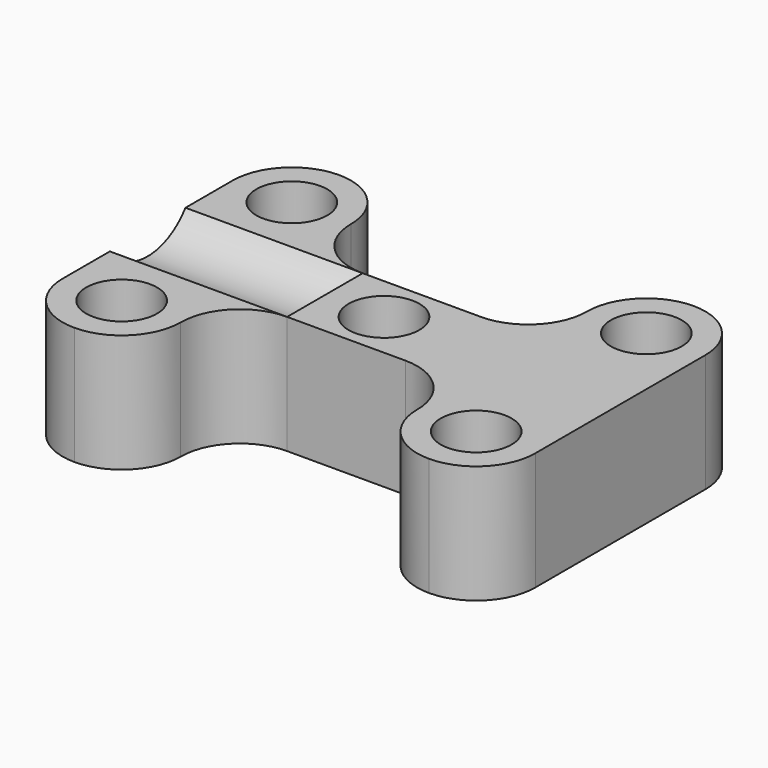
from build123d import *

# Parameters (mm, degrees)
F1_W       = 10
F1_H       = 10
F2_DEPTH   = 10
F1_H_2     = 8
F1_W_2     = 20
F3_DEPTH   = 10
F5_DEPTH   = 15
F6_D       = 6
F6_DEPTH   = 20
F6_TIP     = 1.8025818571
F6_2_D     = 6
F6_2_DEPTH = 20
F6_2_TIP   = 1.8025818571
F6_3_D     = 6
F6_3_DEPTH = 20
F6_3_TIP   = 1.8025818571
F6_4_D     = 6
F6_4_DEPTH = 20
F6_4_TIP   = 1.8025818571
F6_5_D     = 6
F6_5_DEPTH = 20
F6_5_TIP   = 1.8025818571
F7_R       = 5
F7_2_R     = 5
F7_3_R     = 5
F7_4_R     = 5
F9_R       = 4.99999


# Not quite as in the source:
# - a fillet or chamfer is up to 0.001 mm smaller than in the source, because OpenCascade refuses the exact size


with BuildPart() as f2:
    # F1 (on Top) → F2 (new body)
    with BuildSketch(Plane.XY):
        with Locations((-20, -1.6993483007)):
            Rectangle(F1_W, F1_H)
    extrude(amount=F2_DEPTH)

    # F6
    with Locations(Plane(origin=(0, 0, 0), x_dir=(1, 0, 0), z_dir=(0, 0, -1))):
        with Locations((-20, 1.6993483007), (-5, 10.6993483007), (10, 1.6993483007), (10, 19.6993483007), (-20, 19.6993483007)):
            Hole(F6_D / 2, depth=F6_DEPTH)
            with Locations((0, 0, -(F6_DEPTH + F6_TIP / 2))):  # 118° drill point
                Cone(0, F6_D / 2, F6_TIP, mode=Mode.SUBTRACT)

    # F7
    f7_edges = [f2.edges().sort_by_distance(p)[0] for p in [
        (-25, 3.300652, 5),
    ]]
    fillet(f7_edges, radius=F7_R)


with BuildPart() as f2b:
    # F1 (on Top) → F2, piece 2 (new body)
    with BuildSketch(Plane.XY):
        with Locations((-20, -19.6993483007)):
            Rectangle(F1_W, F1_H)
    extrude(amount=F2_DEPTH)

    # F6#2
    with Locations(Plane(origin=(0, 0, 0), x_dir=(1, 0, 0), z_dir=(0, 0, -1))):
        with Locations((-20, 1.6993483007), (-5, 10.6993483007), (10, 1.6993483007), (10, 19.6993483007), (-20, 19.6993483007)):
            Hole(F6_2_D / 2, depth=F6_2_DEPTH)
            with Locations((0, 0, -(F6_2_DEPTH + F6_2_TIP / 2))):  # 118° drill point
                Cone(0, F6_2_D / 2, F6_2_TIP, mode=Mode.SUBTRACT)

    # F7#2
    f7_2_edges = [f2b.edges().sort_by_distance(p)[0] for p in [
        (-25, -24.699348, 5),
    ]]
    fillet(f7_2_edges, radius=F7_2_R)


with BuildPart() as f2c:
    # F1 (on Top) → F2, piece 3 (new body)
    with BuildSketch(Plane.XY):
        with Locations((10, -1.6993483007)):
            Rectangle(F1_W, F1_H)
    extrude(amount=F2_DEPTH)

    # F6#3
    with Locations(Plane(origin=(0, 0, 0), x_dir=(1, 0, 0), z_dir=(0, 0, -1))):
        with Locations((-20, 1.6993483007), (-5, 10.6993483007), (10, 1.6993483007), (10, 19.6993483007), (-20, 19.6993483007)):
            Hole(F6_3_D / 2, depth=F6_3_DEPTH)
            with Locations((0, 0, -(F6_3_DEPTH + F6_3_TIP / 2))):  # 118° drill point
                Cone(0, F6_3_D / 2, F6_3_TIP, mode=Mode.SUBTRACT)

    # F7#4
    f7_4_edges = [f2c.edges().sort_by_distance(p)[0] for p in [
        (15, 3.300652, 5),
    ]]
    fillet(f7_4_edges, radius=F7_4_R)


with BuildPart() as f2d:
    # F1 (on Top) → F2, piece 4 (new body)
    with BuildSketch(Plane.XY):
        with Locations((10, -19.6993483007)):
            Rectangle(F1_W, F1_H)
    extrude(amount=F2_DEPTH)

    # F6#4
    with Locations(Plane(origin=(0, 0, 0), x_dir=(1, 0, 0), z_dir=(0, 0, -1))):
        with Locations((-20, 1.6993483007), (-5, 10.6993483007), (10, 1.6993483007), (10, 19.6993483007), (-20, 19.6993483007)):
            Hole(F6_4_D / 2, depth=F6_4_DEPTH)
            with Locations((0, 0, -(F6_4_DEPTH + F6_4_TIP / 2))):  # 118° drill point
                Cone(0, F6_4_D / 2, F6_4_TIP, mode=Mode.SUBTRACT)

    # F7#3
    f7_3_edges = [f2d.edges().sort_by_distance(p)[0] for p in [
        (15, -24.699348, 5),
    ]]
    fillet(f7_3_edges, radius=F7_3_R)


with BuildPart() as f3:
    # F1 (on Top) → F3 (new body)
    with BuildSketch(Plane.XY):
        with Locations((-20, -10.6993483007)):
            Rectangle(F1_W, F1_H_2)
        with Locations((-5, -10.6993483007)):
            Rectangle(F1_W_2, F1_H_2)
        with Locations((10, -10.6993483007)):
            Rectangle(F1_W, F1_H_2)
    extrude(amount=F3_DEPTH)

    # F4 (on face) → F5 (cut)
    with BuildSketch(Plane(origin=(-25, 0, 0), x_dir=(0, -1, 0), z_dir=(-1, 0, 0))):
        with BuildLine():
            Line((14.6993483007, 10), (6.6993483007, 10))
            ThreePointArc((6.6993483007, 10), (10.6993483007, 8), (14.6993483007, 10))
        make_face()
    extrude(amount=-F5_DEPTH, mode=Mode.SUBTRACT)

    # F6#5
    with Locations(Plane(origin=(0, 0, 0), x_dir=(1, 0, 0), z_dir=(0, 0, -1))):
        with Locations((-20, 1.6993483007), (-5, 10.6993483007), (10, 1.6993483007), (10, 19.6993483007), (-20, 19.6993483007)):
            Hole(F6_5_D / 2, depth=F6_5_DEPTH)
            with Locations((0, 0, -(F6_5_DEPTH + F6_5_TIP / 2))):  # 118° drill point
                Cone(0, F6_5_D / 2, F6_5_TIP, mode=Mode.SUBTRACT)


with BuildPart() as f2_1:
    add(f2.part)

    # F8: union F2c, F3, F2b, F2d
    add(f2c.part)
    add(f3.part)
    add(f2b.part)
    add(f2d.part)

    # F9 (radius 5 in the source; OpenCascade refuses exactly that, so slightly less here)
    f9_edges = [f2_1.edges().sort_by_distance(p)[0] for p in [
        (-15, 3.300652, 5),
        (5, 3.300652, 5),
        (-15, -24.699348, 5),
        (5, -24.699348, 5),
        (-15, -14.699348, 5),
        (5, -14.699348, 5),
        (5, -6.699348, 5),
        (-15, -6.699348, 5),
    ]]
    fillet(f9_edges, radius=F9_R)


solid = f2_1.part
